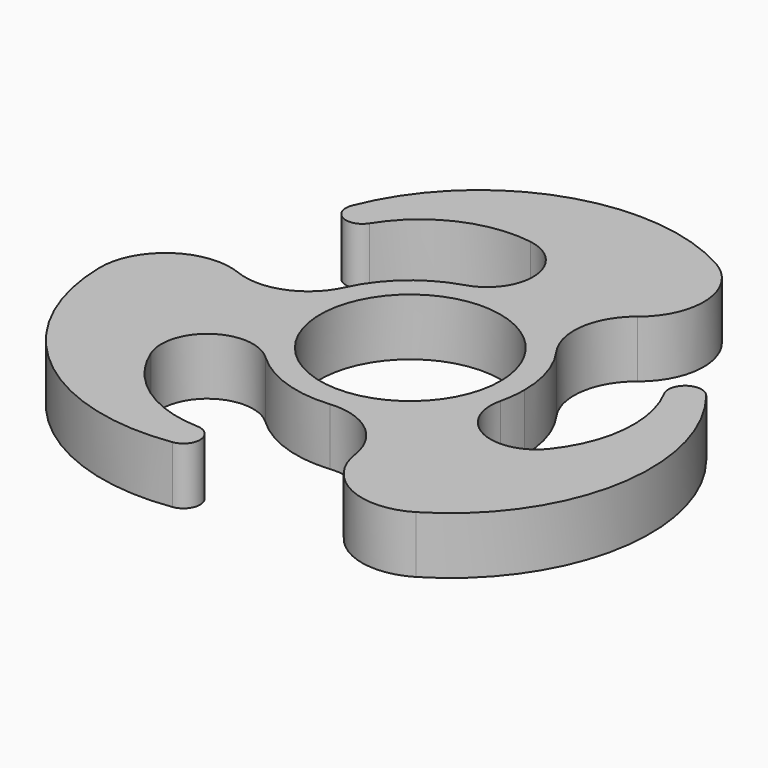
from build123d import *

# Parameters (mm, degrees)
F0_R     = 11.05
F1_DEPTH = 7


# Not quite as in the source:
# - a feature names something its author has since deleted; it is built from what else it names


with BuildPart() as f1:
    # F0 (on Top) → F1 (new body)
    with BuildSketch(Plane.XY):
        with BuildLine():
            ThreePointArc((-4.0106673609, 13.4132228536), (4.561996815, 13.2358673709), (11.4233995183, 8.0935742071))
            ThreePointArc((11.4233995183, 8.0935742071), (10.0789971933, 13.6745719731), (12.9496720608, 18.6459077574))
            ThreePointArc((12.9496720608, 18.6459077574), (15.9741224369, 25.5738093143), (11.8787878788, 31.9276549937))
            ThreePointArc((11.8787878788, 31.9276549937), (-8.2529606774, 33.568130398), (-22.7753295029, 19.5296382006))
            ThreePointArc((-22.7753295029, 19.5296382006), (-21.7981073273, 16.9621679379), (-19.1543041216, 17.7086070442))
            ThreePointArc((-19.1543041216, 17.7086070442), (-12.9655505969, 23.1890748663), (-4.7818295921, 24.3565114828))
            ThreePointArc((-4.7818295921, 24.3565114828), (-0.0139046539, 19.1936864048), (-4.0106673609, 13.4132228536))
        make_face()
        with BuildLine():
            ThreePointArc((13.6215254183, -3.2332716061), (13.9050594363, -1.6276738223), (14, 0))
            ThreePointArc((14, 0), (13.3403072164, 4.2469051522), (11.4233995183, 8.0935742071))
            ThreePointArc((11.4233995183, 8.0935742071), (4.561996815, 13.2358673709), (-4.0106673609, 13.4132228536))
            ThreePointArc((-4.0106673609, 13.4132228536), (-9.1815989768, 10.5687388192), (-12.7209406299, 5.8461670769))
            ThreePointArc((-12.7209406299, 5.8461670769), (-13.7435957918, -2.6671285517), (-9.6108580574, -10.1799512475))
            ThreePointArc((-9.6108580574, -10.1799512475), (-4.561996815, -13.2358673709), (1.2975411116, -13.939741284))
            ThreePointArc((1.2975411116, -13.939741284), (9.1815989768, -10.5687388192), (13.6215254183, -3.2332716061))
        make_face()
        Circle(F0_R, mode=Mode.SUBTRACT)
        with BuildLine():
            ThreePointArc((-9.6108580574, -10.1799512475), (-13.7435957918, -2.6671285517), (-12.7209406299, 5.8461670769))
            ThreePointArc((-12.7209406299, 5.8461670769), (-16.8820253112, 1.8913816276), (-22.6226658249, 1.8917910967))
            ThreePointArc((-22.6226658249, 1.8917910967), (-30.1346297562, 1.0470911764), (-33.5895542472, -5.6764954277))
            ThreePointArc((-33.5895542472, -5.6764954277), (-24.9443733435, -23.931338802), (-5.5254980569, -29.4888330294))
            ThreePointArc((-5.5254980569, -29.4888330294), (-3.7906146738, -27.3587986688), (-5.7589515051, -25.4424174832))
            ThreePointArc((-5.7589515051, -25.4424174832), (-13.5995526261, -22.8230336242), (-18.7024428957, -16.3194416447))
            ThreePointArc((-18.7024428957, -16.3194416447), (-16.6152676918, -9.6088849859), (-9.6108580574, -10.1799512475))
        make_face()
        with BuildLine():
            ThreePointArc((23.4842724877, -8.0370698381), (16.6291723457, -9.5848014189), (13.6215254183, -3.2332716061))
            ThreePointArc((13.6215254183, -3.2332716061), (9.1815989768, -10.5687388192), (1.2975411116, -13.939741284))
            ThreePointArc((1.2975411116, -13.939741284), (6.8030281179, -15.5659536006), (9.6729937641, -20.537698854))
            ThreePointArc((9.6729937641, -20.537698854), (14.1605073193, -26.6209004907), (21.7107663685, -26.2511595661))
            ThreePointArc((21.7107663685, -26.2511595661), (33.1973340209, -9.6367915959), (28.3008275599, 9.9591948288))
            ThreePointArc((28.3008275599, 9.9591948288), (25.5887220011, 10.3966307309), (24.9132556267, 7.733810439))
            ThreePointArc((24.9132556267, 7.733810439), (26.565103223, -0.3660412422), (23.4842724877, -8.0370698381))
        make_face()
    extrude(amount=F1_DEPTH)


solid = f1.part
